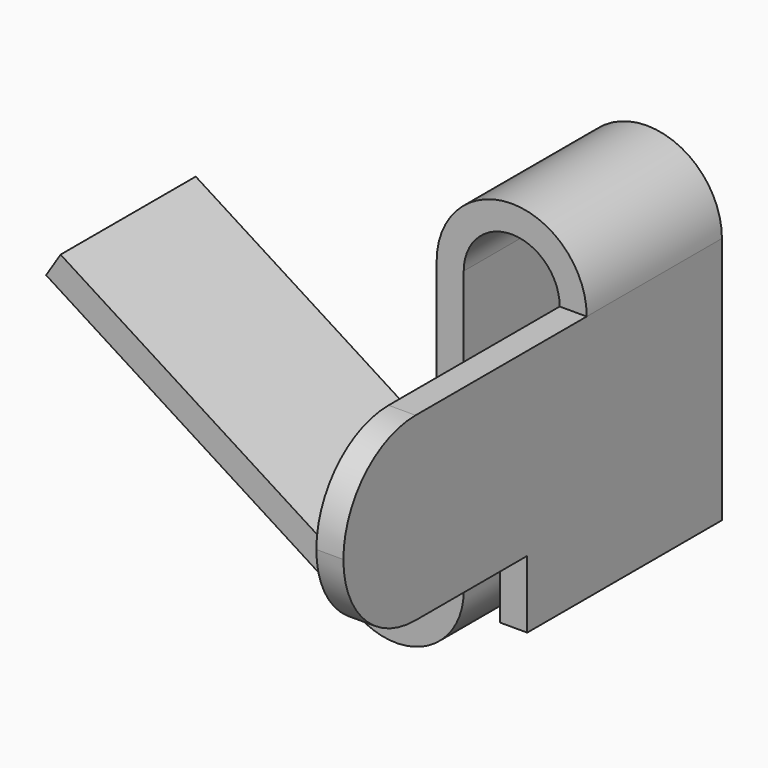
from build123d import *

# Parameters (mm, degrees)
F1_DEPTH = 2.5
F2_W     = 0.4
F2_H     = 3.67
F3_DEPTH = 4.5
F4_W     = 3.4
F4_H     = 1
F5_DEPTH = 25
F6_R     = 1.33499


# Not quite as in the source:
# - a fillet or chamfer is up to 0.001 mm smaller than in the source, because OpenCascade refuses the exact size
# - ends of sketch curves that miss each other by under 0.0002 mm in the source are joined


with BuildPart() as f1:
    # F0 (on Front) → F1 (new body)
    with BuildSketch(Plane.XZ):
        with BuildLine():
            Line((0.71, 1.835), (0.71, -1.835))
            Line((0.71, -1.835), (1.11, -1.835))
            Line((1.11, -1.835), (1.11, 1.835))
            ThreePointArc((1.11, 1.835), (0, 2.945), (-1.11, 1.835))
            Line((-1.11, 1.835), (-1.11, -2.3328240747))
            ThreePointArc((-1.11, -2.3328240747), (-1.421083088, -2.8586837383), (-2.031758919, -2.8392524256))
            Line((-2.031758919, -2.8392524256), (-6.6740188024, 0.1102260326))
            Line((-6.6740188024, 0.1102260326), (-6.8885263266, -0.227392868))
            Line((-6.8885263266, -0.227392868), (-2.2462664432, -3.1768713262))
            ThreePointArc((-2.2462664432, -3.1768713262), (-1.2294272033, -3.2097802095), (-0.71, -2.335))
            Line((-0.71, -2.335), (-0.71, 1.835))
            ThreePointArc((-0.71, 1.835), (0, 2.545), (0.71, 1.835))
        make_face()
    extrude(amount=F1_DEPTH)

    # F2 (on face) → F3 (join)
    with BuildSketch(Plane.XZ.offset(2.5)):
        with Locations((0.91, 0)):
            Rectangle(F2_W, F2_H)
    extrude(amount=F3_DEPTH)

    # F4 (on face) → F5 (cut)
    with BuildSketch(Plane.YZ.offset(1.11)):
        with Locations((-5.3, -1.335)):
            Rectangle(F4_W, F4_H)
    extrude(amount=-F5_DEPTH, mode=Mode.SUBTRACT)

    # F6 (radius 1.335 in the source; OpenCascade refuses exactly that, so slightly less here)
    f6_edges = [f1.edges().sort_by_distance(p)[0] for p in [
        (0.91, -7, 1.835),
        (0.91, -7, -0.835),
    ]]
    fillet(f6_edges, radius=F6_R)


solid = f1.part
